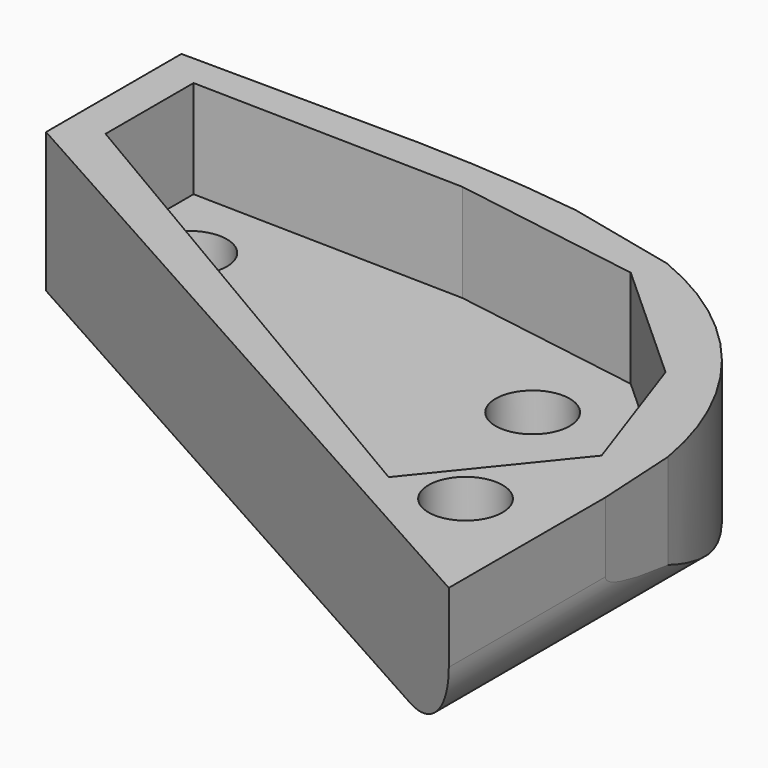
from build123d import *

# Parameters (mm, degrees)
F1_DEPTH    = 10
F2_R        = 2.65
F2_R_2      = 2.7
F3_DEPTH    = 10.001
F4_T1_DEPTH = 74
F6_DEPTH    = 7


# Not quite as in the source:
# - a fillet or chamfer that OpenCascade refuses, or shapes differently, is made with other operations: its cross-section is extruded or revolved along the edge and cut away or added


with BuildPart() as f1:
    # F0 (on Top) → F1 (new body)
    with BuildSketch(Plane.XY):
        with BuildLine():
            Line((-33.8368600405, -9.2521366523), (-50.8368600405, -9.1521366523))
            Line((-50.8368600405, -9.1521366523), (-50.8368600405, -21.2521366523))
            Line((-50.8368600405, -21.2521366523), (1.1631399595, -50.2521366523))
            Line((1.1631399595, -50.2521366523), (1.1631399595, -36.2521366523))
            Line((1.1631399595, -36.2521366523), (0.8274590919, -30.2521366523))
            ThreePointArc((0.8274590919, -30.2521366523), (-4.1287803642, -19.2185823544), (-13.8368600405, -12.003541191))
            Line((-13.8368600405, -12.003541191), (-21.8368600405, -10.1521366523))
            ThreePointArc((-21.8368600405, -10.1521366523), (-27.8233098501, -9.521467447), (-33.8368600405, -9.2521366523))
        make_face()
    extrude(amount=F1_DEPTH)

    # F2 (on face) → F3 (cut, through all)
    with BuildSketch(Plane.XY.offset(10)):
        with Locations((-43.8368600405, -17.1521366523)):
            Circle(F2_R)
        with Locations((-16.8368600405, -20.2521366523)):
            Circle(F2_R)
        with Locations((-4.8368600405, -41.2521366523)):
            Circle(F2_R)
        with Locations((-10.8368600405, -29.2521366523)):
            Circle(F2_R_2)
    extrude(amount=-F3_DEPTH, mode=Mode.SUBTRACT)

    # F4: fillet of radius 5 on 1 edges, made by hand

    # F4_s2 → F4_t1 (cut)
    with BuildSketch(Plane.XZ.offset(6.2521366523)):
        with BuildLine():
            ThreePointArc((-3.8368600405, 0), (-0.3013261345, 1.4644660941), (1.1631399595, 5))
            Line((1.1631399595, 5), (1.2631399595, 5))
            Line((1.2631399595, 5), (1.2631399595, -0.1))
            Line((1.2631399595, -0.1), (-3.8368600405, -0.1))
            Line((-3.8368600405, -0.1), (-3.8368600405, 0))
        make_face()
    extrude(amount=F4_T1_DEPTH, mode=Mode.SUBTRACT)

    # F5 (on face) → F6 (cut)
    with BuildSketch(Plane.XY.offset(10)):
        Polygon((-28.5395178944, -11.904838495), (-48.1065809727, -11.4794680849), (-48.1065809727, -19.3488299847), (-9.8231984302, -41.8934859335), (-2.166522434, -32.4289835989), (-5.6758336723, -22.3264265805), (-14.7149646655, -14.1380364075), align=None)
    extrude(amount=-F6_DEPTH, mode=Mode.SUBTRACT)


solid = f1.part
